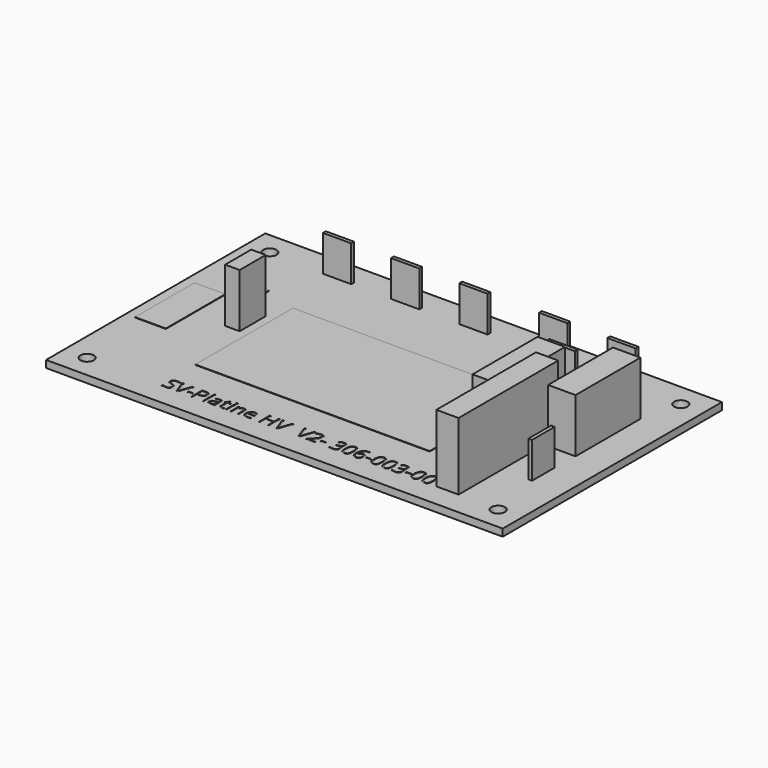
from build123d import *

# Parameters (mm, degrees)
F0_W         = 101.6
F0_H         = 60.96
F0_R         = 1.5
F0_W_2       = 6.8493969738
F0_H_2       = 16.5560217574
F0_W_3       = 52.1439313889
F0_H_3       = 27.1404888481
F0_W_4       = 4.9363300204
F0_H_4       = 27.7038663626
F0_W_5       = 0.8
F0_H_5       = 6.3
F0_W_6       = 3.2237172127
F0_H_6       = 7.2533756029
F0_W_7       = 2.54
F0_H_7       = 5.08
F0_W_8       = 6.3
F0_H_8       = 0.8
F0_W_9       = 6.0948543251
F0_H_9       = 18.0830685422
F0_W_10      = 6.0993358493
F0_H_10      = 18.043874763
F1_DEPTH     = 1.6
F2_TEXT_SIZE = 4.3633388633
F3_DEPTH     = 0.1
F4_DEPTH     = 8
F5_DEPTH     = 12
F6_DEPTH     = 15
F7_DEPTH     = 0.1


# Not quite as in the source:
# - Text() gives the source's letters only with a copy of the font that has no kerning and outlines rounded to 1/6400 em; it was checked with that copy


with BuildPart() as f1:
    # F0 (on Top) → F1 (new body)
    with BuildSketch(Plane.XY):
        Rectangle(F0_W, F0_H)
        with Locations((-45.72, -25.4)):
            Circle(F0_R, mode=Mode.SUBTRACT)
        with Locations((-45.2461522073, -0.1165899448)):
            Rectangle(F0_W_2, F0_H_2, mode=Mode.SUBTRACT)
        with Locations((-3.2858625054, -2.2011669353)):
            Rectangle(F0_W_3, F0_H_3, mode=Mode.SUBTRACT)
        with Locations((45.72, -25.4)):
            Circle(F0_R, mode=Mode.SUBTRACT)
        with Locations((34.3505777419, -11.4337801933)):
            Rectangle(F0_W_4, F0_H_4, mode=Mode.SUBTRACT)
        with Locations((43.1330576539, -10.1021388546)):
            Rectangle(F0_W_5, F0_H_5, mode=Mode.SUBTRACT)
        with Locations((-32.8806601465, 2.5702770799)):
            Rectangle(F0_W_6, F0_H_6, mode=Mode.SUBTRACT)
        with Locations((-38.0024759877, 11.3860016996)):
            Rectangle(F0_W_7, F0_H_7, mode=Mode.SUBTRACT)
        with Locations((-45.72, 25.4)):
            Circle(F0_R, mode=Mode.SUBTRACT)
        with Locations((-30.3416382521, 25.2782758325)):
            Rectangle(F0_W_8, F0_H_8, mode=Mode.SUBTRACT)
        with Locations((-15.1885375381, 25.2782758325)):
            Rectangle(F0_W_8, F0_H_8, mode=Mode.SUBTRACT)
        with Locations((0, 25.2782758325)):
            Rectangle(F0_W_8, F0_H_8, mode=Mode.SUBTRACT)
        with Locations((27.9005076736, 2.6058219373)):
            Rectangle(F0_W_9, F0_H_9, mode=Mode.SUBTRACT)
        with Locations((40.6475737691, 7.6690060087)):
            Rectangle(F0_W_10, F0_H_10, mode=Mode.SUBTRACT)
        with Locations((25.3358229488, 17.8651667476)):
            Rectangle(F0_W_8, F0_H_8, mode=Mode.SUBTRACT)
        with Locations((17.7241396159, 25.2782758325)):
            Rectangle(F0_W_8, F0_H_8, mode=Mode.SUBTRACT)
        with Locations((32.9301282763, 25.2782758325)):
            Rectangle(F0_W_8, F0_H_8, mode=Mode.SUBTRACT)
        with Locations((45.72, 25.4)):
            Circle(F0_R, mode=Mode.SUBTRACT)
        with Locations((-45.2461522073, -0.1165899448)):
            Rectangle(F0_W_2, F0_H_2)
        with Locations((-32.8806601465, 2.5702770799)):
            Rectangle(F0_W_6, F0_H_6)
        with Locations((-3.2858625054, -2.2011669353)):
            Rectangle(F0_W_3, F0_H_3)
        with Locations((27.9005076736, 2.6058219373)):
            Rectangle(F0_W_9, F0_H_9)
        with Locations((34.3505777419, -11.4337801933)):
            Rectangle(F0_W_4, F0_H_4)
        with Locations((40.6475737691, 7.6690060087)):
            Rectangle(F0_W_10, F0_H_10)
        with Locations((-30.3416382521, 25.2782758325)):
            Rectangle(F0_W_8, F0_H_8)
        with Locations((-15.1885375381, 25.2782758325)):
            Rectangle(F0_W_8, F0_H_8)
        with Locations((0, 25.2782758325)):
            Rectangle(F0_W_8, F0_H_8)
        with Locations((17.7241396159, 25.2782758325)):
            Rectangle(F0_W_8, F0_H_8)
        with Locations((32.9301282763, 25.2782758325)):
            Rectangle(F0_W_8, F0_H_8)
        with Locations((25.3358229488, 17.8651667476)):
            Rectangle(F0_W_8, F0_H_8)
        with Locations((43.1330576539, -10.1021388546)):
            Rectangle(F0_W_5, F0_H_5)
        with Locations((-38.0024759877, 11.3860016996)):
            Rectangle(F0_W_7, F0_H_7)
    extrude(amount=-F1_DEPTH)

    # F2 (on face) → F3 (cut)
    with BuildSketch(Plane.XY):
        with Locations((-29.2592132554, -25.6216039815)):
            Text('SV-Platine HV  V2- 306-003-00', F2_TEXT_SIZE, font='Open Sans', text_align=(TextAlign.LEFT, TextAlign.BOTTOM))
    extrude(amount=-F3_DEPTH, mode=Mode.SUBTRACT)

    # F0 (on Top) → F5 (join)
    with BuildSketch(Plane.XY):
        with Locations((27.9005076736, 2.6058219373)):
            Rectangle(F0_W_9, F0_H_9)
        with Locations((40.6475737691, 7.6690060087)):
            Rectangle(F0_W_10, F0_H_10)
        with Locations((-32.8806601465, 2.5702770799)):
            Rectangle(F0_W_6, F0_H_6)
    extrude(amount=F5_DEPTH)

    # F0 (on Top) → F7 (join)
    with BuildSketch(Plane.XY):
        with Locations((-45.2461522073, -0.1165899448)):
            Rectangle(F0_W_2, F0_H_2)
        with Locations((-38.0024759877, 11.3860016996)):
            Rectangle(F0_W_7, F0_H_7)
        with Locations((-3.2858625054, -2.2011669353)):
            Rectangle(F0_W_3, F0_H_3)
    extrude(amount=F7_DEPTH)


with BuildPart() as f4:
    # F0 (on Top) → F4 (new body)
    with BuildSketch(Plane.XY):
        with Locations((0, 25.2782758325)):
            Rectangle(F0_W_8, F0_H_8)
    extrude(amount=F4_DEPTH)


with BuildPart() as f4b:
    # F0 (on Top) → F4, piece 2 (new body)
    with BuildSketch(Plane.XY):
        with Locations((17.7241396159, 25.2782758325)):
            Rectangle(F0_W_8, F0_H_8)
    extrude(amount=F4_DEPTH)


with BuildPart() as f4c:
    # F0 (on Top) → F4, piece 3 (new body)
    with BuildSketch(Plane.XY):
        with Locations((32.9301282763, 25.2782758325)):
            Rectangle(F0_W_8, F0_H_8)
    extrude(amount=F4_DEPTH)


with BuildPart() as f4d:
    # F0 (on Top) → F4, piece 4 (new body)
    with BuildSketch(Plane.XY):
        with Locations((25.3358229488, 17.8651667476)):
            Rectangle(F0_W_8, F0_H_8)
    extrude(amount=F4_DEPTH)


with BuildPart() as f4e:
    # F0 (on Top) → F4, piece 5 (new body)
    with BuildSketch(Plane.XY):
        with Locations((43.1330576539, -10.1021388546)):
            Rectangle(F0_W_5, F0_H_5)
    extrude(amount=F4_DEPTH)


with BuildPart() as f4f:
    # F0 (on Top) → F4, piece 6 (new body)
    with BuildSketch(Plane.XY):
        with Locations((-15.1885375381, 25.2782758325)):
            Rectangle(F0_W_8, F0_H_8)
    extrude(amount=F4_DEPTH)


with BuildPart() as f4g:
    # F0 (on Top) → F4, piece 7 (new body)
    with BuildSketch(Plane.XY):
        with Locations((-30.3416382521, 25.2782758325)):
            Rectangle(F0_W_8, F0_H_8)
    extrude(amount=F4_DEPTH)


with BuildPart() as f6:
    # F0 (on Top) → F6 (new body)
    with BuildSketch(Plane.XY):
        with Locations((34.3505777419, -11.4337801933)):
            Rectangle(F0_W_4, F0_H_4)
    extrude(amount=F6_DEPTH)


solid = Compound([f1.part, f4.part, f4b.part, f4c.part, f4d.part, f4e.part, f4f.part, f4g.part, f6.part])
